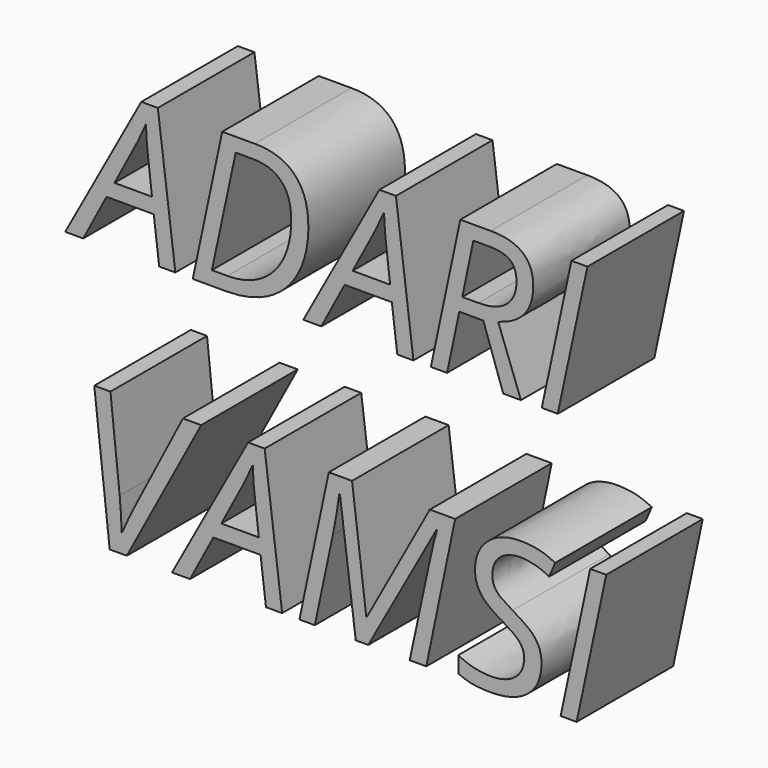
from build123d import *

# Parameters (mm, degrees)
F0_TEXT_SIZE = 40.3743961619
F1_DEPTH     = 25


# Not quite as in the source:
# - Text() gives the source's letters only with a copy of the font that has no kerning and outlines rounded to 1/6400 em; it was checked with that copy


with BuildPart() as f1:
    # F0 (on Front) → F1 (new body)
    with BuildSketch(Plane.XZ):
        with Locations((-57.3284883002, -29.0695652366)):
            Text('ADARI', F0_TEXT_SIZE, font='Open Sans', font_style=FontStyle.ITALIC, text_align=(TextAlign.LEFT, TextAlign.BOTTOM))
        with Locations((-57.3284883002, -83.9787440168)):
            Text('VAMSI', F0_TEXT_SIZE, font='Open Sans', font_style=FontStyle.ITALIC, text_align=(TextAlign.LEFT, TextAlign.BOTTOM))
    extrude(amount=F1_DEPTH)


solid = f1.part
